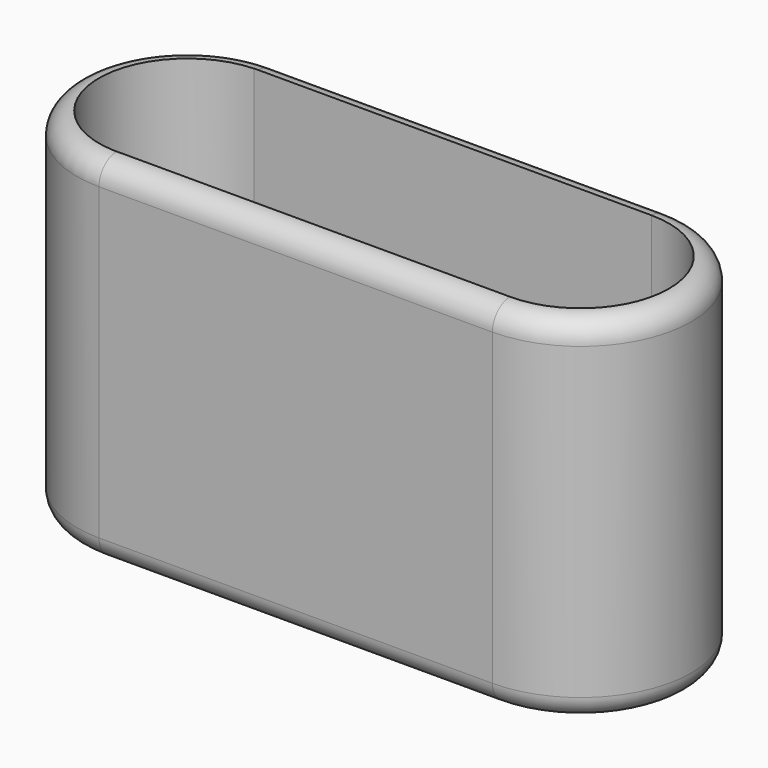
from build123d import *

# Parameters (mm, degrees)
F2_DEPTH    = 80
F3_DEPTH    = 5
F4_W        = 80
F4_H        = 3
F5_DEPTH    = 5
F6_T1_DEPTH = 89.0924813444
F6_T4_ANGLE = 180
F6_T6_ANGLE = 180
F7_T1_DEPTH = 89.0924813444
F7_T4_ANGLE = 180
F7_T6_ANGLE = 180


# Not quite as in the source:
# - a fillet or chamfer that OpenCascade refuses, or shapes differently, is made with other operations: its cross-section is extruded or revolved along the edge and cut away or added


with BuildPart() as f2:
    # F0 (on Top) → F2 (new body)
    with BuildSketch(Plane.XY):
        with BuildLine():
            Line((44.6416767532, 25), (-44.4508045912, 25))
            ThreePointArc((-44.4508045912, 25), (-69.4508045912, 0), (-44.4508045912, -25))
            Line((-44.4508045912, -25), (44.6416767532, -25))
            ThreePointArc((44.6416767532, -25), (69.6416767532, 0), (44.6416767532, 25))
        make_face()
        with BuildLine():
            Line((-45.3583232468, 19.9793996379), (-45.3583232468, 20.0206003621))
            Line((-45.3583232468, 20.0206003621), (44.6416767532, 20.0206003621))
            Line((44.6416767532, 20.0206003621), (44.6416767532, 20))
            ThreePointArc((44.6416767532, 20), (64.6365259994, -0.4538762181), (43.7341580975, -19.9793996379))
            Line((43.7341580975, -19.9793996379), (-43.5432859355, -19.9793996379))
            ThreePointArc((-43.5432859355, -19.9793996379), (-44.4508045912, -20), (-45.3583232468, -19.9793996379))
            ThreePointArc((-45.3583232468, -19.9793996379), (-64.4508045912, 0), (-45.3583232468, 19.9793996379))
        make_face(mode=Mode.SUBTRACT)
    extrude(amount=F2_DEPTH)

    # F1 (on Top) → F3 (join)
    with BuildSketch(Plane.XY):
        with BuildLine():
            Line((45.1049394906, 20), (-44.8950605094, 20))
            ThreePointArc((-44.8950605094, 20), (-64.8950605094, 0), (-44.8950605094, -20))
            Line((-44.8950605094, -20), (-39.8680716753, -20))
            Line((-39.8680716753, -20), (40.1319283247, -20))
            Line((40.1319283247, -20), (45.1049394906, -20))
            ThreePointArc((45.1049394906, -20), (65.1049394906, 0), (45.1049394906, 20))
        make_face()
    extrude(amount=F3_DEPTH)

    # F4 (on face) → F5 (join)
    with BuildSketch(Plane.XY.offset(5)):
        with Locations((0.1319283247, -1.5)):
            Rectangle(F4_W, F4_H)
    extrude(amount=F5_DEPTH)

    # F6: fillet of radius 5 on 1 edges, made by hand

    # F6_s2 → F6_t1 (cut)
    with BuildSketch(Plane.YZ.offset(-44.4508045912)):
        with BuildLine():
            ThreePointArc((-20, 80), (-23.5355339059, 78.5355339059), (-25, 75))
            Line((-25, 75), (-25, 80))
            Line((-25, 80), (-20, 80))
        make_face()
        with BuildLine():
            ThreePointArc((25, 75), (23.5355339059, 78.5355339059), (20, 80))
            Line((20, 80), (25, 80))
            Line((25, 80), (25, 75))
        make_face()
    extrude(amount=F6_T1_DEPTH, mode=Mode.SUBTRACT)

    # F6_s3 → F6_t4 (revolve, cut)
    with BuildSketch(Plane.YZ.offset(-44.4508045912)):
        with BuildLine():
            ThreePointArc((25, 75), (23.5355339059, 78.5355339059), (20, 80))
            Line((20, 80), (25, 80))
            Line((25, 80), (25, 75))
        make_face()
    revolve(axis=Axis((-44.4508045912, 0, 80), (0, 0, 1)), revolution_arc=F6_T4_ANGLE, mode=Mode.SUBTRACT)

    # F6_s5 → F6_t6 (revolve, cut)
    with BuildSketch(Plane.YZ.offset(44.6416767532)):
        with BuildLine():
            ThreePointArc((-25, 75), (-23.5355339059, 78.5355339059), (-20, 80))
            Line((-20, 80), (-25, 80))
            Line((-25, 80), (-25, 75))
        make_face()
    revolve(axis=Axis((44.6416767532, 0, 80), (0, 0, 1)), revolution_arc=F6_T6_ANGLE, mode=Mode.SUBTRACT)

    # F7: fillet of radius 5 on 5 edges, made by hand

    # F7_s2 → F7_t1 (cut)
    with BuildSketch(Plane.YZ.offset(-44.4508045912)):
        with BuildLine():
            ThreePointArc((-20, 0), (-23.5355339059, 1.4644660941), (-25, 5))
            Line((-25, 5), (-25, 0))
            Line((-25, 0), (-20, 0))
        make_face()
        with BuildLine():
            ThreePointArc((25, 5), (23.5355339059, 1.4644660941), (20, 0))
            Line((20, 0), (25, 0))
            Line((25, 0), (25, 5))
        make_face()
    extrude(amount=F7_T1_DEPTH, mode=Mode.SUBTRACT)

    # F7_s3 → F7_t4 (revolve, cut)
    with BuildSketch(Plane.YZ.offset(-44.4508045912)):
        with BuildLine():
            ThreePointArc((20, 0), (23.5355339059, 1.4644660941), (25, 5))
            Line((25, 5), (25, 0))
            Line((25, 0), (20, 0))
        make_face()
    revolve(axis=Axis((-44.4508045912, 0, 0), (0, 0, 1)), revolution_arc=F7_T4_ANGLE, mode=Mode.SUBTRACT)

    # F7_s5 → F7_t6 (revolve, cut)
    with BuildSketch(Plane.YZ.offset(44.6416767532)):
        with BuildLine():
            ThreePointArc((-20, 0), (-23.5355339059, 1.4644660941), (-25, 5))
            Line((-25, 5), (-25, 0))
            Line((-25, 0), (-20, 0))
        make_face()
    revolve(axis=Axis((44.6416767532, 0, 0), (0, 0, 1)), revolution_arc=F7_T6_ANGLE, mode=Mode.SUBTRACT)


solid = f2.part
